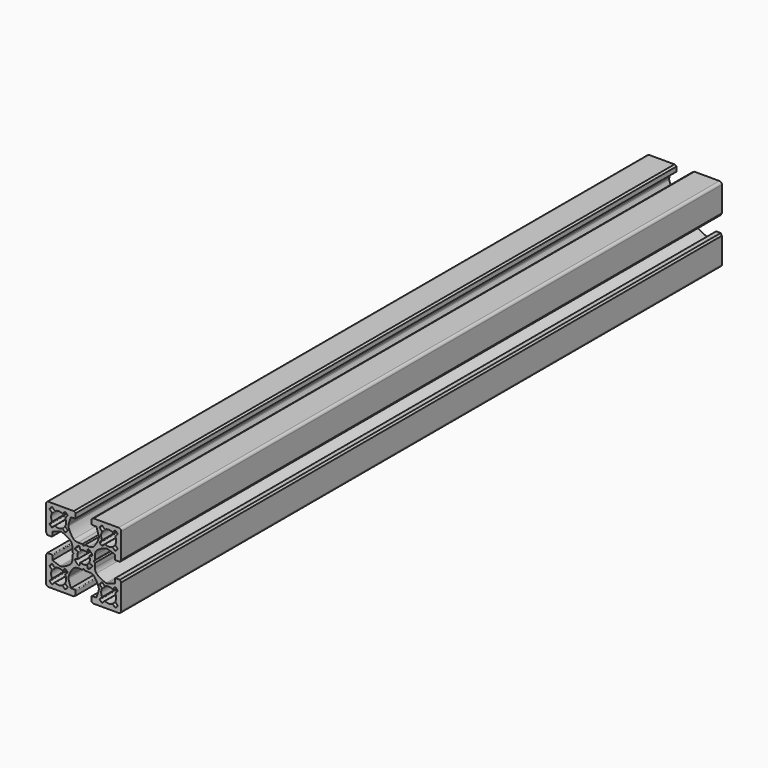
from build123d import *

# Parameters (mm, degrees)
F1_DEPTH = 300


# Not quite as in the source:
# - ends of sketch curves that miss each other by under 0.0002 mm in the source are joined


with BuildPart() as f1:
    # F0 (on Front) → F1 (new body)
    with BuildSketch(Plane.XZ):
        with BuildLine():
            Line((-16.817882, -28.053804), (-15.317882, -28.053804))
            ThreePointArc((-15.317882, -28.053804), (-15.2613573135, -27.5251941322), (-15.0943392862, -27.0204878701))
            ThreePointArc((-15.0943392862, -27.0204878701), (-15.1018556445, -26.757114112), (-15.3142900125, -26.6012490693))
            Line((-15.3142900125, -26.6012490693), (-16.055223, -26.467679))
            ThreePointArc((-16.055223, -26.467679), (-16.2747726412, -26.2973161033), (-16.2602657097, -26.0198001716))
            ThreePointArc((-16.2602657097, -26.0198001716), (-15.6451391247, -25.2265468753), (-14.8518861678, -24.611419716))
            ThreePointArc((-14.8518861678, -24.611419716), (-14.574370128, -24.5969122529), (-14.4040070693, -24.8164620125))
            Line((-14.4040070693, -24.8164620125), (-14.270436, -25.557396))
            ThreePointArc((-14.270436, -25.557396), (-14.114570705, -25.7698304515), (-13.8511966819, -25.7773467007))
            ThreePointArc((-13.8511966819, -25.7773467007), (-13.3464912208, -25.6103285465), (-12.817882, -25.553804))
            Line((-12.817882, -25.553804), (-12.817882, -24.053804))
            Line((-12.817882, -24.053804), (-13.317882, -23.553804))
            Line((-13.317882, -23.553804), (-15.035723, -23.553804))
            ThreePointArc((-15.035723, -23.553804), (-15.9762206131, -23.4025693887), (-16.8218943655, -22.9641134932))
            ThreePointArc((-16.8218943655, -22.9641134932), (-18.0925440917, -21.1637239049), (-18.9312372647, -19.1259440756))
            ThreePointArc((-18.9312372647, -19.1259440756), (-18.952848093, -18.864054156), (-18.9054896298, -18.6055767962))
            Line((-18.9054896298, -18.6055767962), (-17.917882, -15.553804))
            Line((-17.917882, -15.553804), (-16.267882, -15.553804))
            ThreePointArc((-16.267882, -15.553804), (-16.0557499656, -15.4659360344), (-15.967882, -15.253804))
            Line((-15.967882, -15.253804), (-15.967882, -13.553804))
            Line((-15.967882, -13.553804), (-16.767882, -13.053804))
            Line((-16.767882, -13.053804), (-26.817882, -13.053804))
            ThreePointArc((-26.817882, -13.053804), (-27.5249887812, -13.3466972188), (-27.817882, -14.053804))
            Line((-27.817882, -14.053804), (-27.817882, -24.103804))
            Line((-27.817882, -24.103804), (-27.317882, -24.903804))
            Line((-27.317882, -24.903804), (-25.617882, -24.903804))
            ThreePointArc((-25.617882, -24.903804), (-25.4057499656, -24.8159360344), (-25.317882, -24.603804))
            Line((-25.317882, -24.603804), (-25.317882, -22.953804))
            Line((-25.317882, -22.953804), (-22.266108, -21.966196))
            ThreePointArc((-22.266108, -21.966196), (-22.0076307271, -21.9188378518), (-21.7457409226, -21.9404486442))
            ThreePointArc((-21.7457409226, -21.9404486442), (-19.7079616374, -22.7791421598), (-17.907572504, -24.049791567))
            ThreePointArc((-17.907572504, -24.049791567), (-17.4691166439, -24.8954652882), (-17.317882, -25.835963))
            Line((-17.317882, -25.835963), (-17.317882, -27.553804))
            Line((-17.317882, -27.553804), (-16.817882, -28.053804))
        make_face()
        with BuildLine():
            ThreePointArc((-20.1318415243, -16.7176952608), (-19.817882, -18.053804), (-20.1318415243, -19.3899127392))
            ThreePointArc((-20.1318415243, -19.3899127392), (-20.1593135799, -19.5718836819), (-20.0753690344, -19.7356560344))
            Line((-20.0753690344, -19.7356560344), (-19.334799, -20.476227))
            ThreePointArc((-19.334799, -20.476227), (-19.2473630595, -20.6722640002), (-19.3132911489, -20.8765408801))
            ThreePointArc((-19.3132911489, -20.8765408801), (-19.6359009875, -21.2357840182), (-19.9951440617, -21.5583939234))
            ThreePointArc((-19.9951440617, -21.5583939234), (-20.1994212978, -21.6243229782), (-20.3954590344, -21.5368870344))
            Line((-20.3954590344, -21.5368870344), (-21.136029, -20.796316))
            ThreePointArc((-21.136029, -20.796316), (-21.2998015274, -20.7123715492), (-21.4817721923, -20.7398436134))
            ThreePointArc((-21.4817721923, -20.7398436134), (-22.8178815523, -21.053804), (-24.153991138, -20.7398442773))
            ThreePointArc((-24.153991138, -20.7398442773), (-24.3359616819, -20.7123714201), (-24.4997340344, -20.7963159656))
            Line((-24.4997340344, -20.7963159656), (-25.240304, -21.536887))
            ThreePointArc((-25.240304, -21.536887), (-25.4363417022, -21.6243229782), (-25.6406189751, -21.5583939691))
            ThreePointArc((-25.6406189751, -21.5583939691), (-25.9998625153, -21.2357845153), (-26.322472412, -20.8765413318))
            ThreePointArc((-26.322472412, -20.8765413318), (-26.3884009573, -20.6722643134), (-26.3009650344, -20.4762269656))
            Line((-26.3009650344, -20.4762269656), (-25.560394, -19.735656))
            ThreePointArc((-25.560394, -19.735656), (-25.4764494201, -19.5718836819), (-25.5039220121, -19.389913006))
            ThreePointArc((-25.5039220121, -19.389913006), (-25.817882, -18.053804), (-25.5039222773, -16.717694862))
            ThreePointArc((-25.5039222773, -16.717694862), (-25.4764494201, -16.5357243181), (-25.5603939656, -16.3719519656))
            Line((-25.5603939656, -16.3719519656), (-26.300965, -15.631381))
            ThreePointArc((-26.300965, -15.631381), (-26.3884009573, -15.4353436866), (-26.3224724576, -15.2310666314))
            ThreePointArc((-26.3224724576, -15.2310666314), (-25.9998625153, -14.8718234847), (-25.6406193318, -14.549213588))
            ThreePointArc((-25.6406193318, -14.549213588), (-25.4363417022, -14.4832850218), (-25.2403039656, -14.5707209656))
            Line((-25.2403039656, -14.5707209656), (-24.499734, -15.311292))
            ThreePointArc((-24.499734, -15.311292), (-24.3359616819, -15.3952365799), (-24.153991006, -15.3677639879))
            ThreePointArc((-24.153991006, -15.3677639879), (-22.8178815523, -15.053804), (-21.4817720604, -15.3677641214))
            ThreePointArc((-21.4817720604, -15.3677641214), (-21.2998015274, -15.3952364508), (-21.1360294656, -15.3112915344))
            Line((-21.1360294656, -15.3112915344), (-20.395459, -14.570721))
            ThreePointArc((-20.395459, -14.570721), (-20.1994212978, -14.4832850218), (-19.9951440249, -14.5492140309))
            ThreePointArc((-19.9951440249, -14.5492140309), (-19.6359009875, -14.8718239818), (-19.3132911946, -15.2310671567))
            ThreePointArc((-19.3132911946, -15.2310671567), (-19.2473630595, -15.4353439998), (-19.3347989656, -15.6313810344))
            Line((-19.3347989656, -15.6313810344), (-20.075369, -16.371952))
            ThreePointArc((-20.075369, -16.371952), (-20.1593135799, -16.5357243181), (-20.1318415243, -16.7176952608))
        make_face(mode=Mode.SUBTRACT)
        with BuildLine():
            Line((-10.317882, -28.053804), (-8.817882, -28.053804))
            Line((-8.817882, -28.053804), (-8.317882, -27.553804))
            Line((-8.317882, -27.553804), (-8.317882, -25.835963))
            ThreePointArc((-8.317882, -25.835963), (-8.1666472628, -24.8954650055), (-7.7281910149, -24.049790989))
            ThreePointArc((-7.7281910149, -24.049790989), (-5.9278016138, -22.7791417483), (-3.8900220756, -21.9404487353))
            ThreePointArc((-3.8900220756, -21.9404487353), (-3.6281322729, -21.9188378518), (-3.3696549943, -21.9661959825))
            Line((-3.3696549943, -21.9661959825), (-0.317882, -22.953804))
            Line((-0.317882, -22.953804), (-0.317882, -24.603804))
            ThreePointArc((-0.317882, -24.603804), (-0.2300140344, -24.8159360344), (-0.017882, -24.903804))
            Line((-0.017882, -24.903804), (1.682118, -24.903804))
            Line((1.682118, -24.903804), (2.182118, -24.103804))
            Line((2.182118, -24.103804), (2.182118, -14.053804))
            ThreePointArc((2.182118, -14.053804), (1.8892247812, -13.3466972188), (1.182118, -13.053804))
            Line((1.182118, -13.053804), (-8.867882, -13.053804))
            Line((-8.867882, -13.053804), (-9.667882, -13.553804))
            Line((-9.667882, -13.553804), (-9.667882, -15.253804))
            ThreePointArc((-9.667882, -15.253804), (-9.5800140344, -15.4659360344), (-9.367882, -15.553804))
            Line((-9.367882, -15.553804), (-7.717882, -15.553804))
            Line((-7.717882, -15.553804), (-6.730274, -18.605577))
            ThreePointArc((-6.730274, -18.605577), (-6.6829159047, -18.8640542036), (-6.7045263914, -19.1259439149))
            ThreePointArc((-6.7045263914, -19.1259439149), (-7.5432189083, -21.1637239049), (-8.8138685119, -22.9641134339))
            ThreePointArc((-8.8138685119, -22.9641134339), (-9.6595430055, -23.4025692628), (-10.600041, -23.553804))
            Line((-10.600041, -23.553804), (-12.317882, -23.553804))
            Line((-12.317882, -23.553804), (-12.817882, -24.053804))
            Line((-12.817882, -24.053804), (-12.817882, -25.553804))
            ThreePointArc((-12.817882, -25.553804), (-12.2892723342, -25.6103286428), (-11.7845662465, -25.777346543))
            ThreePointArc((-11.7845662465, -25.777346543), (-11.521192295, -25.7698304515), (-11.3653270693, -25.5573959875))
            Line((-11.3653270693, -25.5573959875), (-11.231756, -24.816462))
            ThreePointArc((-11.231756, -24.816462), (-11.061392872, -24.5969122529), (-10.7838767336, -24.6114195492))
            ThreePointArc((-10.7838767336, -24.6114195492), (-9.990624391, -25.2265473595), (-9.3754974572, -26.0198002702))
            ThreePointArc((-9.3754974572, -26.0198002702), (-9.3609903588, -26.2973161033), (-9.5805400125, -26.4676789307))
            Line((-9.5805400125, -26.4676789307), (-10.321473, -26.601249))
            ThreePointArc((-10.321473, -26.601249), (-10.5339073555, -26.757114112), (-10.5414238716, -27.0204879417))
            ThreePointArc((-10.5414238716, -27.0204879417), (-10.3744066428, -27.5251943342), (-10.317882, -28.053804))
        make_face()
        with BuildLine():
            ThreePointArc((-5.5627339656, -19.7356560344), (-5.4787894201, -19.5718836819), (-5.5062620121, -19.389913006))
            ThreePointArc((-5.5062620121, -19.389913006), (-5.820221, -18.053804), (-5.5062614757, -16.7176952608))
            ThreePointArc((-5.5062614757, -16.7176952608), (-5.4787894201, -16.5357243181), (-5.5627339656, -16.3719519656))
            Line((-5.5627339656, -16.3719519656), (-6.303305, -15.631381))
            ThreePointArc((-6.303305, -15.631381), (-6.3907399595, -15.4353436467), (-6.3248118511, -15.2310671199))
            ThreePointArc((-6.3248118511, -15.2310671199), (-6.0022020125, -14.8718239818), (-5.6429589383, -14.5492140766))
            ThreePointArc((-5.6429589383, -14.5492140766), (-5.4386817022, -14.4832850218), (-5.2426439656, -14.5707209656))
            Line((-5.2426439656, -14.5707209656), (-4.502074, -15.311292))
            ThreePointArc((-4.502074, -15.311292), (-4.3383016819, -15.3952365799), (-4.156331006, -15.3677639879))
            ThreePointArc((-4.156331006, -15.3677639879), (-2.8202214477, -15.053804), (-1.484111862, -15.3677637227))
            ThreePointArc((-1.484111862, -15.3677637227), (-1.3021413181, -15.3952365799), (-1.1383689656, -15.3112920344))
            Line((-1.1383689656, -15.3112920344), (-0.397799, -14.570721))
            ThreePointArc((-0.397799, -14.570721), (-0.2017612978, -14.4832850218), (0.0025159751, -14.5492140309))
            ThreePointArc((0.0025159751, -14.5492140309), (0.3617595153, -14.8718234847), (0.684369412, -15.2310666682))
            ThreePointArc((0.684369412, -15.2310666682), (0.7502979573, -15.4353436866), (0.6628620344, -15.6313810344))
            Line((0.6628620344, -15.6313810344), (-0.077709, -16.371952))
            ThreePointArc((-0.077709, -16.371952), (-0.1616535799, -16.5357243181), (-0.1341809879, -16.717694994))
            ThreePointArc((-0.1341809879, -16.717694994), (0.179779, -18.053804), (-0.1341807227, -19.389913138))
            ThreePointArc((-0.1341807227, -19.389913138), (-0.1616535799, -19.5718836819), (-0.0777090344, -19.7356560344))
            Line((-0.0777090344, -19.7356560344), (0.662862, -20.476227))
            ThreePointArc((0.662862, -20.476227), (0.7502979573, -20.6722643134), (0.6843694576, -20.8765413686))
            ThreePointArc((0.6843694576, -20.8765413686), (0.3617595153, -21.2357845153), (0.0025163318, -21.558394412))
            ThreePointArc((0.0025163318, -21.558394412), (-0.2017612978, -21.6243229782), (-0.3977990344, -21.5368870344))
            Line((-0.3977990344, -21.5368870344), (-1.138369, -20.796316))
            ThreePointArc((-1.138369, -20.796316), (-1.3021413181, -20.7123714201), (-1.484111994, -20.7398440121))
            ThreePointArc((-1.484111994, -20.7398440121), (-2.8202214477, -21.053804), (-4.1563309396, -20.7398438786))
            ThreePointArc((-4.1563309396, -20.7398438786), (-4.3383016819, -20.7123714201), (-4.5020740344, -20.7963159656))
            Line((-4.5020740344, -20.7963159656), (-5.242644, -21.536887))
            ThreePointArc((-5.242644, -21.536887), (-5.4386817022, -21.6243229782), (-5.6429589751, -21.5583939691))
            ThreePointArc((-5.6429589751, -21.5583939691), (-6.0022020125, -21.2357840182), (-6.3248118054, -20.8765408433))
            ThreePointArc((-6.3248118054, -20.8765408433), (-6.3907399595, -20.6722643533), (-6.3033045344, -20.4762274656))
            Line((-6.3033045344, -20.4762274656), (-5.5627339656, -19.7356560344))
        make_face(mode=Mode.SUBTRACT)
        with BuildLine():
            Line((-8.317882, -28.553804), (-8.817882, -28.053804))
            Line((-8.817882, -28.053804), (-10.317882, -28.053804))
            ThreePointArc((-10.317882, -28.053804), (-10.3744066428, -28.5824136658), (-10.541424543, -29.0871197535))
            ThreePointArc((-10.541424543, -29.0871197535), (-10.5339073967, -29.3504938095), (-10.3214731621, -29.5063588992))
            Line((-10.3214731621, -29.5063588992), (-9.58054, -29.639929))
            ThreePointArc((-9.58054, -29.639929), (-9.3609903588, -29.8102918967), (-9.3754972903, -30.0878078284))
            ThreePointArc((-9.3754972903, -30.0878078284), (-9.990624391, -30.8810606405), (-10.783877091, -31.496187846))
            ThreePointArc((-10.783877091, -31.496187846), (-11.061392872, -31.5106957471), (-11.2317559307, -31.2911459875))
            Line((-11.2317559307, -31.2911459875), (-11.365327, -30.550212))
            ThreePointArc((-11.365327, -30.550212), (-11.521192112, -30.3377776445), (-11.7845659417, -30.3302611284))
            ThreePointArc((-11.7845659417, -30.3302611284), (-12.2892721322, -30.4972793135), (-12.817882, -30.553804))
            Line((-12.817882, -30.553804), (-12.817882, -32.053804))
            Line((-12.817882, -32.053804), (-12.317882, -32.553804))
            Line((-12.317882, -32.553804), (-10.600041, -32.553804))
            ThreePointArc((-10.600041, -32.553804), (-9.6595430055, -32.7050387372), (-8.813868989, -33.1434949851))
            ThreePointArc((-8.813868989, -33.1434949851), (-7.5432189083, -34.9438840951), (-6.7045257353, -36.9816639244))
            ThreePointArc((-6.7045257353, -36.9816639244), (-6.6829158812, -37.2435533212), (-6.7302739825, -37.5020300057))
            Line((-6.7302739825, -37.5020300057), (-7.717882, -40.553804))
            Line((-7.717882, -40.553804), (-9.367882, -40.553804))
            ThreePointArc((-9.367882, -40.553804), (-9.5800140344, -40.6416719656), (-9.667882, -40.853804))
            Line((-9.667882, -40.853804), (-9.667882, -42.553804))
            Line((-9.667882, -42.553804), (-8.867882, -43.053804))
            Line((-8.867882, -43.053804), (1.182118, -43.053804))
            ThreePointArc((1.182118, -43.053804), (1.8892247812, -42.7609107812), (2.182118, -42.053804))
            Line((2.182118, -42.053804), (2.182118, -32.003804))
            Line((2.182118, -32.003804), (1.682118, -31.203804))
            Line((1.682118, -31.203804), (-0.017882, -31.203804))
            ThreePointArc((-0.017882, -31.203804), (-0.2300140344, -31.2916719656), (-0.317882, -31.503804))
            Line((-0.317882, -31.503804), (-0.317882, -33.153804))
            Line((-0.317882, -33.153804), (-3.369655, -34.141412))
            ThreePointArc((-3.369655, -34.141412), (-3.6281322729, -34.1887701482), (-3.8900220774, -34.1671593558))
            ThreePointArc((-3.8900220774, -34.1671593558), (-5.9278016138, -33.3284662517), (-7.7281909374, -32.0578169295))
            ThreePointArc((-7.7281909374, -32.0578169295), (-8.1666472628, -31.2121429945), (-8.317882, -30.271645))
            Line((-8.317882, -30.271645), (-8.317882, -28.553804))
        make_face()
        with BuildLine():
            ThreePointArc((-5.507146239, -39.3904841188), (-5.8210019909, -38.0543501064), (-5.5069379006, -36.7182650494))
            ThreePointArc((-5.5069379006, -36.7182650494), (-5.4794506299, -36.5362965287), (-5.5633824662, -36.3725174663))
            Line((-5.5633824662, -36.3725174663), (-6.303896, -35.631889))
            ThreePointArc((-6.303896, -35.631889), (-6.3913162338, -35.4358449105), (-6.3253716664, -35.2315732687))
            ThreePointArc((-6.3253716664, -35.2315732687), (-6.0027340882, -34.8723550769), (-5.6434657786, -34.5497732749))
            ThreePointArc((-5.6434657786, -34.5497732749), (-5.4391833549, -34.483860277), (-5.2431524662, -34.5713114663))
            Line((-5.2431524662, -34.5713114663), (-4.50264, -35.31194))
            ThreePointArc((-4.50264, -35.31194), (-4.3388740212, -35.3958977668), (-4.1569008286, -35.3684393446))
            ThreePointArc((-4.1569008286, -35.3684393446), (-2.8207674361, -35.0545840092), (-1.4846830494, -35.3686480994))
            ThreePointArc((-1.4846830494, -35.3686480994), (-1.3027146578, -35.3961343911), (-1.1389359663, -35.3122030337))
            Line((-1.1389359663, -35.3122030337), (-0.398307, -34.57169))
            ThreePointArc((-0.398307, -34.57169), (-0.2022626922, -34.4842688081), (0.0020096134, -34.5502132386))
            ThreePointArc((0.0020096134, -34.5502132386), (0.3612269231, -34.8728519118), (0.6838087251, -35.2321202214))
            ThreePointArc((0.6838087251, -35.2321202214), (0.7497216831, -35.4364023869), (0.6622700337, -35.6324330337))
            Line((0.6622700337, -35.6324330337), (-0.078358, -36.372946))
            ThreePointArc((-0.078358, -36.372946), (-0.1623158238, -36.5367113277), (-0.1348573446, -36.7186841714))
            ThreePointArc((-0.1348573446, -36.7186841714), (0.1789979909, -38.0548178935), (-0.1350659009, -39.3909025518))
            ThreePointArc((-0.1350659009, -39.3909025518), (-0.162552241, -39.5728712621), (-0.0786200338, -39.7366500338))
            Line((-0.0786200338, -39.7366500338), (0.661893, -40.477278))
            ThreePointArc((0.661893, -40.477278), (0.7493132149, -40.6733227364), (0.6833686664, -40.8775947313))
            ThreePointArc((0.6833686664, -40.8775947313), (0.3607308072, -41.2368122042), (0.0014628737, -41.5593938432))
            ThreePointArc((0.0014628737, -41.5593938432), (-0.202819292, -41.625306742), (-0.3988500338, -41.5378560338))
            Line((-0.3988500338, -41.5378560338), (-1.139363, -40.797227))
            ThreePointArc((-1.139363, -40.797227), (-1.303129108, -40.7132702121), (-1.4851017727, -40.7407284571))
            ThreePointArc((-1.4851017727, -40.7407284571), (-2.8212354459, -41.0545839909), (-4.157320149, -40.7405202994))
            ThreePointArc((-4.157320149, -40.7405202994), (-4.3392886912, -40.7130336658), (-4.5030675338, -40.7969654663))
            Line((-4.5030675338, -40.7969654663), (-5.243696, -41.537478))
            ThreePointArc((-5.243696, -41.537478), (-5.4397403476, -41.624898194), (-5.6440121248, -41.5589541549))
            ThreePointArc((-5.6440121248, -41.5589541549), (-6.0032304261, -41.2363165853), (-6.3258123317, -40.8770482671))
            ThreePointArc((-6.3258123317, -40.8770482671), (-6.3917246831, -40.6727656131), (-6.3042730337, -40.4767349663))
            Line((-6.3042730337, -40.4767349663), (-5.563645, -39.736222))
            ThreePointArc((-5.563645, -39.736222), (-5.4796873054, -39.5724564631), (-5.507146239, -39.3904841188))
        make_face(mode=Mode.SUBTRACT)
        with BuildLine():
            ThreePointArc((-15.0943392862, -29.0871201299), (-15.2613573135, -28.5824138678), (-15.317882, -28.053804))
            Line((-15.317882, -28.053804), (-16.817882, -28.053804))
            Line((-16.817882, -28.053804), (-17.317882, -28.553804))
            Line((-17.317882, -28.553804), (-17.317882, -30.271645))
            ThreePointArc((-17.317882, -30.271645), (-17.4691166439, -31.2121427118), (-17.9075726307, -32.0578165326))
            ThreePointArc((-17.9075726307, -32.0578165326), (-19.7079616374, -33.3284658402), (-21.7457409999, -34.1671590005))
            ThreePointArc((-21.7457409999, -34.1671590005), (-22.0076307271, -34.1887701482), (-22.2661080057, -34.1414120175))
            Line((-22.2661080057, -34.1414120175), (-25.317882, -33.153804))
            Line((-25.317882, -33.153804), (-25.317882, -31.503804))
            ThreePointArc((-25.317882, -31.503804), (-25.4057499656, -31.2916719656), (-25.617882, -31.203804))
            Line((-25.617882, -31.203804), (-27.317882, -31.203804))
            Line((-27.317882, -31.203804), (-27.817882, -32.003804))
            Line((-27.817882, -32.003804), (-27.817882, -42.053804))
            ThreePointArc((-27.817882, -42.053804), (-27.5249887812, -42.7609107812), (-26.817882, -43.053804))
            Line((-26.817882, -43.053804), (-16.767882, -43.053804))
            Line((-16.767882, -43.053804), (-15.967882, -42.553804))
            Line((-15.967882, -42.553804), (-15.967882, -40.853804))
            ThreePointArc((-15.967882, -40.853804), (-16.0557499656, -40.6416719656), (-16.267882, -40.553804))
            Line((-16.267882, -40.553804), (-17.917882, -40.553804))
            Line((-17.917882, -40.553804), (-18.905489, -37.50203))
            ThreePointArc((-18.905489, -37.50203), (-18.9528481165, -37.2435533689), (-18.9312375634, -36.9816638775))
            ThreePointArc((-18.9312375634, -36.9816638775), (-18.0925440917, -34.9438840951), (-16.8218944881, -33.1434945661))
            ThreePointArc((-16.8218944881, -33.1434945661), (-15.9762206131, -32.7050386113), (-15.035723, -32.553804))
            Line((-15.035723, -32.553804), (-13.317882, -32.553804))
            Line((-13.317882, -32.553804), (-12.817882, -32.053804))
            Line((-12.817882, -32.053804), (-12.817882, -30.553804))
            ThreePointArc((-12.817882, -30.553804), (-13.3464914228, -30.4972794098), (-13.8511973007, -30.3302616625))
            ThreePointArc((-13.8511973007, -30.3302616625), (-14.114570888, -30.3377776445), (-14.2704359307, -30.5502120125))
            Line((-14.2704359307, -30.5502120125), (-14.404007, -31.291146))
            ThreePointArc((-14.404007, -31.291146), (-14.574370128, -31.5106957471), (-14.8518862664, -31.4961884508))
            ThreePointArc((-14.8518862664, -31.4961884508), (-15.6451391247, -30.8810611247), (-16.260266284, -30.0878081678))
            ThreePointArc((-16.260266284, -30.0878081678), (-16.2747726412, -29.8102918967), (-16.0552229875, -29.6399290693))
            Line((-16.0552229875, -29.6399290693), (-15.31429, -29.506358))
            ThreePointArc((-15.31429, -29.506358), (-15.1018556033, -29.3504938095), (-15.0943392862, -29.0871201299))
        make_face()
        with BuildLine():
            ThreePointArc((-20.0747205338, -36.3725174663), (-20.1586523342, -36.5362963089), (-20.1311656295, -36.7182648157))
            ThreePointArc((-20.1311656295, -36.7182648157), (-19.8171020091, -38.0543498837), (-20.1309575628, -39.3904837201))
            ThreePointArc((-20.1309575628, -39.3904837201), (-20.1584156946, -39.5724564631), (-20.0744580337, -39.7362220337))
            Line((-20.0744580337, -39.7362220337), (-19.33383, -40.476735))
            ThreePointArc((-19.33383, -40.476735), (-19.2463783169, -40.6727656131), (-19.3122908476, -40.8770481227))
            ThreePointArc((-19.3122908476, -40.8770481227), (-19.6348730769, -41.2363160882), (-19.9940910142, -41.5589539824))
            ThreePointArc((-19.9940910142, -41.5589539824), (-20.1983629105, -41.6248982338), (-20.3944070337, -41.5374780337))
            Line((-20.3944070337, -41.5374780337), (-21.135036, -40.796965))
            ThreePointArc((-21.135036, -40.796965), (-21.2988146578, -40.7130336089), (-21.4807828157, -40.7405203705))
            ThreePointArc((-21.4807828157, -40.7405203705), (-22.8168676587, -41.0545839908), (-24.1530013171, -40.7407286377))
            ThreePointArc((-24.1530013171, -40.7407286377), (-24.334973892, -40.7132702121), (-24.4987395337, -40.7972274662))
            Line((-24.4987395337, -40.7972274662), (-25.239253, -41.537856))
            ThreePointArc((-25.239253, -41.537856), (-25.435283708, -41.625306742), (-25.6395657293, -41.5593936639))
            ThreePointArc((-25.6395657293, -41.5593936639), (-25.99883431, -41.2368127014), (-26.3214719824, -40.8775949858))
            ThreePointArc((-26.3214719824, -40.8775949858), (-26.3874162149, -40.6733227364), (-26.2999955337, -40.4772784662))
            Line((-26.2999955337, -40.4772784662), (-25.559483, -39.73665))
            ThreePointArc((-25.559483, -39.73665), (-25.475550759, -39.5728712621), (-25.5030371701, -39.3909025871))
            ThreePointArc((-25.5030371701, -39.3909025871), (-25.8171019909, -38.0548178936), (-25.503246239, -36.7186838812))
            ThreePointArc((-25.503246239, -36.7186838812), (-25.4757871762, -36.5367113277), (-25.5597444663, -36.3729454662))
            Line((-25.5597444663, -36.3729454662), (-26.300374, -35.632433))
            ThreePointArc((-26.300374, -35.632433), (-26.3878247021, -35.4364020339), (-26.3219121524, -35.2321198773))
            ThreePointArc((-26.3219121524, -35.2321198773), (-25.9993304261, -34.8728514147), (-25.6401123794, -34.550213529))
            ThreePointArc((-25.6401123794, -34.550213529), (-25.4358403078, -34.4842688081), (-25.2397959662, -34.5716899662))
            Line((-25.2397959662, -34.5716899662), (-24.499168, -35.312203))
            ThreePointArc((-24.499168, -35.312203), (-24.3353886912, -35.3961343342), (-24.1534201843, -35.3686476295))
            ThreePointArc((-24.1534201843, -35.3686476295), (-22.8173356686, -35.0545840091), (-21.4812022799, -35.3684395628))
            ThreePointArc((-21.4812022799, -35.3684395628), (-21.2992289788, -35.3958977668), (-21.1354629663, -35.3119400337))
            Line((-21.1354629663, -35.3119400337), (-20.39495, -34.571312))
            ThreePointArc((-20.39495, -34.571312), (-20.1989200339, -34.4838602979), (-19.9946378773, -34.5497728476))
            ThreePointArc((-19.9946378773, -34.5497728476), (-19.63536969, -34.8723552987), (-19.312731624, -35.2315735027))
            ThreePointArc((-19.312731624, -35.2315735027), (-19.2467867662, -35.4358449105), (-19.3342069663, -35.6318890337))
            Line((-19.3342069663, -35.6318890337), (-20.0747205338, -36.3725174663))
        make_face(mode=Mode.SUBTRACT)
    extrude(amount=F1_DEPTH)


solid = f1.part
